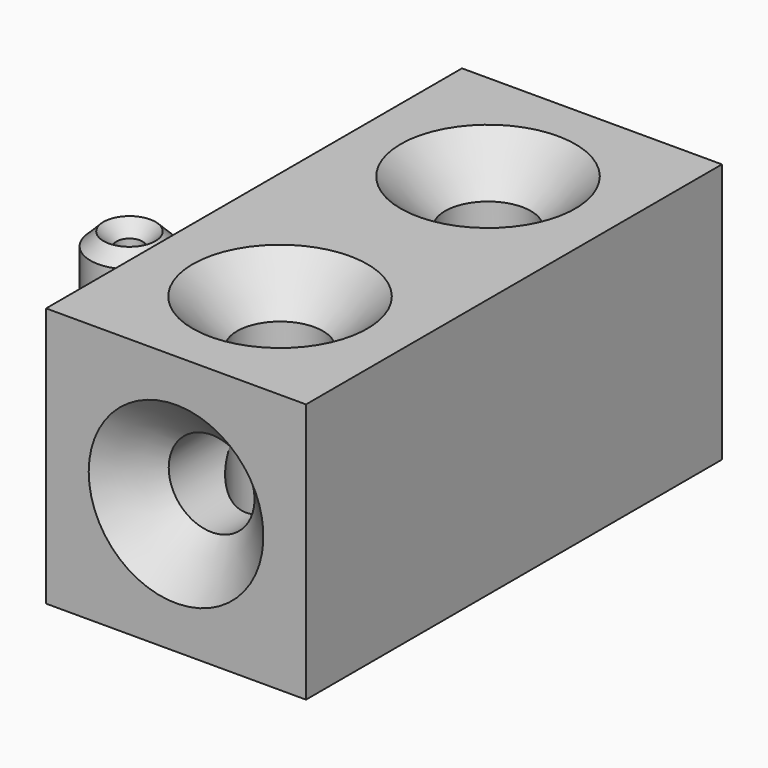
from build123d import *

# Parameters (mm, degrees)
F1_R           = 1.5
F1_R_2         = 0.5
F2_DEPTH       = 3
F3_SIZE        = 0.49999
F4_W           = 10
F4_H           = 20
F5_DEPTH       = 10
F7_D           = 3.3
F7_CSINK_D     = 6.72
F7_CSINK_ANGLE = 90
F9_D           = 3.3
F9_CSINK_D     = 6.72
F9_CSINK_ANGLE = 90


# Not quite as in the source:
# - a fillet or chamfer is up to 0.001 mm smaller than in the source, because OpenCascade refuses the exact size


with BuildPart() as f2:
    # F1 (on Top) → F2 (new body)
    with BuildSketch(Plane.XY):
        Circle(F1_R)
        Circle(F1_R_2, mode=Mode.SUBTRACT)
    extrude(amount=F2_DEPTH)

    # F3 (size 0.5 in the source; OpenCascade refuses exactly that, so slightly less here)
    f3_edges = [f2.edges().sort_by_distance(p)[0] for p in [
        (-0.5, 0, 3),
        (-1.5, 0, 3),
        (-1.5, 0, 0),
        (-0.5, 0, 0),
    ]]
    chamfer(f3_edges, length=F3_SIZE)


with BuildPart() as f5:
    # F4 (on Top) → F5 (new body)
    with BuildSketch(Plane.XY):
        with Locations((14.5698995329, -5.9731390672)):
            Rectangle(F4_W, F4_H)
    extrude(amount=F5_DEPTH)

    # F7 (through all)
    with Locations(Plane.XZ.offset(15.9731390672)):
        with Locations((14.5698995329, 5)):
            CounterSinkHole(F7_D / 2, F7_CSINK_D / 2, counter_sink_angle=F7_CSINK_ANGLE)

    # F9 (through all)
    with Locations(Plane.XY.offset(10)):
        with Locations((14.5698995329, -10.9731390672), (14.5698995329, -0.9731390672)):
            CounterSinkHole(F9_D / 2, F9_CSINK_D / 2, counter_sink_angle=F9_CSINK_ANGLE)


solid = Compound([f2.part, f5.part])
